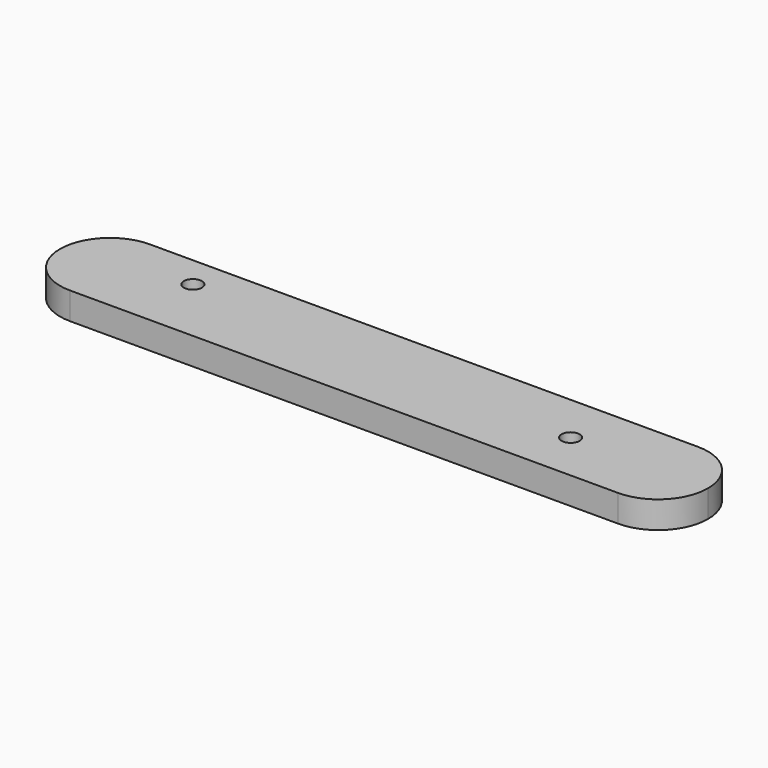
from build123d import *

# Parameters (mm, degrees)
F0_R     = 6.35
F1_DEPTH = 19.05
F2_R     = 35.17899


# Not quite as in the source:
# - a fillet or chamfer is up to 0.001 mm smaller than in the source, because OpenCascade refuses the exact size


with BuildPart() as f1:
    # F0 (on Top) → F1 (new body)
    with BuildSketch(Plane.XY):
        with BuildLine():
            Line((372.999, 22.479), (-48.26, 22.479))
            ThreePointArc((-48.26, 22.479), (-83.439, -12.7), (-48.26, -47.879))
            Line((-48.26, -47.879), (372.999, -47.879))
            Line((372.999, -47.879), (372.999, 22.479))
        make_face()
        Circle(F0_R, mode=Mode.SUBTRACT)
        with Locations((276.225, -12.7)):
            Circle(F0_R, mode=Mode.SUBTRACT)
    extrude(amount=F1_DEPTH)

    # F2 (radius 35.179 in the source; OpenCascade refuses exactly that, so slightly less here)
    f2_edges = [f1.edges().sort_by_distance(p)[0] for p in [
        (372.999, -47.879, 9.525),
        (372.999, 22.479, 9.525),
    ]]
    fillet(f2_edges, radius=F2_R)


solid = f1.part
